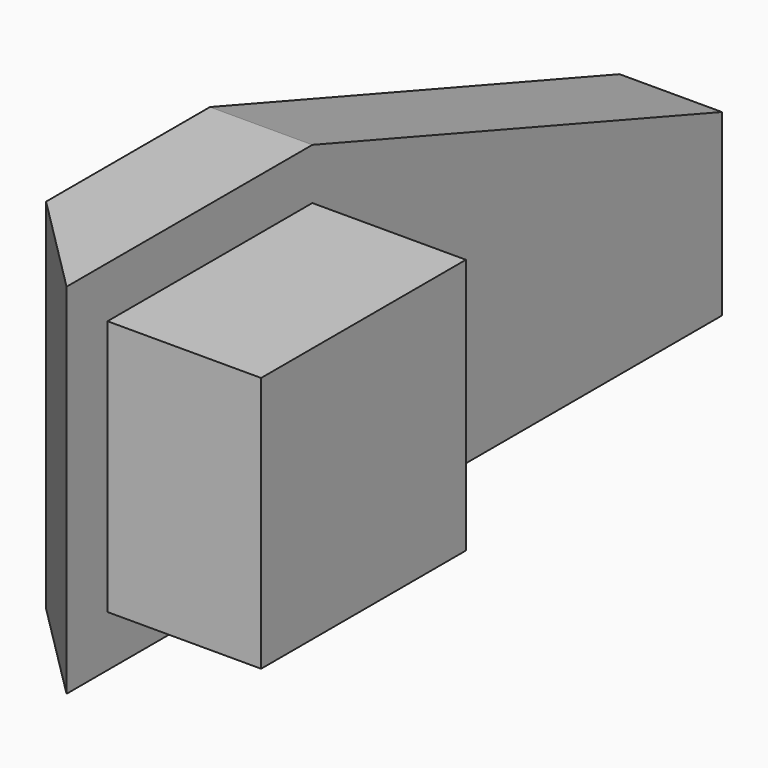
from build123d import *

# Parameters (mm, degrees)
F0_W     = 5
F0_H     = 5
F1_DEPTH = 3
F2_W     = 5
F2_H     = 5
F3_DEPTH = 2
F4_SIZE  = 1.99999


# Not quite as in the source:
# - a fillet or chamfer is up to 0.001 mm smaller than in the source, because OpenCascade refuses the exact size


with BuildPart() as f1:
    # F0 (on Right) → F1 (new body)
    with BuildSketch(Plane.YZ):
        with Locations((40.6040474772, 32.0952650385)):
            Rectangle(F0_W, F0_H)
    extrude(amount=F1_DEPTH)

    # F2 (on face) → F3 (join)
    with BuildSketch(Plane(origin=(0, 0, 0), x_dir=(0, -1, 0), z_dir=(-1, 0, 0))):
        with Locations((-40.6040474772, 32.0952650385)):
            Rectangle(F2_W, F2_H)
        Polygon((-37.1040474772, 28.5952650385), (-37.1040474772, 35.5952650385), (-43.1040474772, 35.5952650385), (-43.1040474772, 34.5952650385), (-38.1040474772, 34.5952650385), (-38.1040474772, 29.5952650385), (-43.1040474772, 29.5952650385), (-43.1040474772, 28.5952650385), align=None)
        Polygon((-43.1040474772, 34.5952650385), (-43.1040474772, 35.5952650385), (-51.1040474772, 32.7952650385), (-51.1040474772, 31.3952650385), (-43.1040474772, 28.5952650385), (-43.1040474772, 29.5952650385), align=None)
        Polygon((-51.1040474772, 31.3952650385), (-51.1040474772, 32.7952650385), (-53.1040474772, 32.0952650385), align=None)
        Polygon((-51.1040474772, 31.3952650385), (-53.1040474772, 32.0952650385), (-53.1040474772, 28.5952650385), (-51.1040474772, 28.5952650385), align=None)
        Polygon((-51.1040474772, 28.5952650385), (-43.1040474772, 28.5952650385), (-51.1040474772, 31.3952650385), align=None)
    extrude(amount=F3_DEPTH)

    # F4 (size 2 in the source; OpenCascade refuses exactly that, so slightly less here)
    f4_edges = [f1.edges().sort_by_distance(p)[0] for p in [
        (-2, 37.104047, 32.095265),
    ]]
    chamfer(f4_edges, length=F4_SIZE)


solid = f1.part
